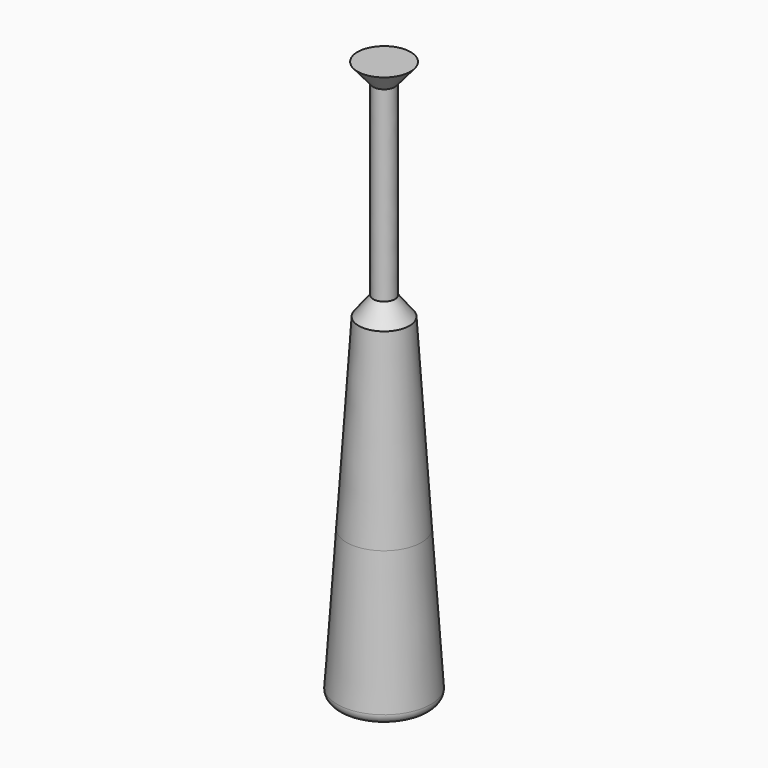
from build123d import *

# Parameters (mm, degrees)
F0_R  = 14.2031372516
F5_R  = 5.7900940223
F6_R  = 5.811478977
F7_R  = 13.5706885585
F8_R  = 20.0607447558
F14_R = 25.3778243108
F16_R = 5


with BuildPart() as f9:
    # F0 (on Top) → F9 section 0
    with BuildSketch(Plane.XY):
        Circle(F0_R)
    # F5 (on offset) → F9 section 1
    with BuildSketch(Plane.XY.offset(-10)):
        Circle(F5_R)
    loft()

    # F5 (on offset) → F10 section 0
    with BuildSketch(Plane.XY.offset(-10)):
        Circle(F5_R)
    # F6 (on offset) → F10 section 1
    with BuildSketch(Plane.XY.offset(-110)):
        Circle(F6_R)
    loft()

    # F6 (on offset) → F11 section 0
    with BuildSketch(Plane.XY.offset(-110)):
        Circle(F6_R)
    # F7 (on offset) → F11 section 1
    with BuildSketch(Plane.XY.offset(-120)):
        Circle(F7_R)
    loft()

    # F7 (on offset) → F12 section 0
    with BuildSketch(Plane.XY.offset(-120)):
        Circle(F7_R)
    # F8 (on offset) → F12 section 1
    with BuildSketch(Plane.XY.offset(-220)):
        Circle(F8_R)
    loft()

    # F8 (on offset) → F15 section 0
    with BuildSketch(Plane.XY.offset(-220)):
        Circle(F8_R)
    # F14 (on offset) → F15 section 1
    with BuildSketch(Plane.XY.offset(-300)):
        Circle(F14_R)
    loft()

    # F16
    f16_edges = [f9.edges().sort_by_distance(p)[0] for p in [
        (-25.377824, 0, -300),
    ]]
    fillet(f16_edges, radius=F16_R)


solid = f9.part
